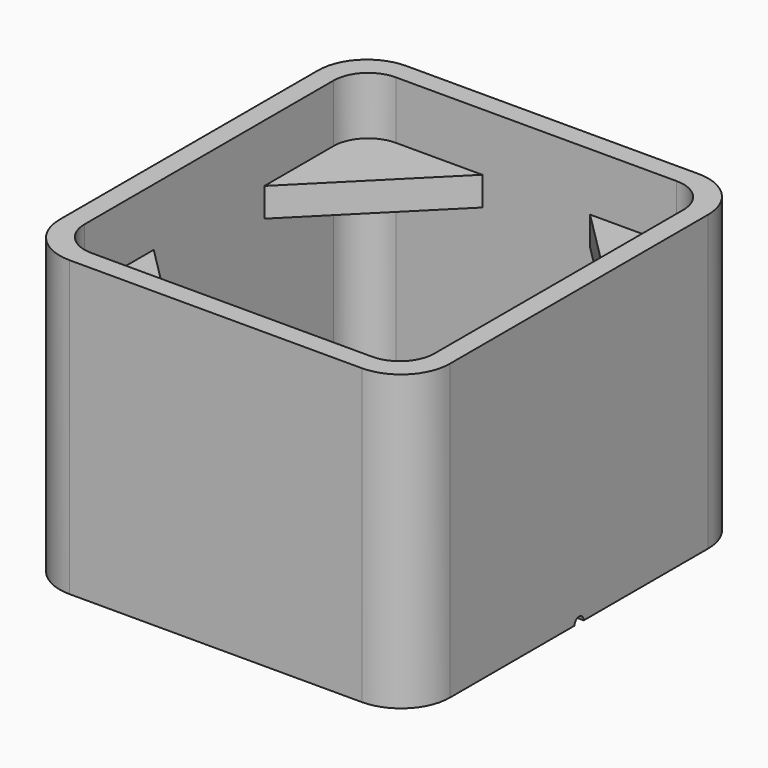
from build123d import *

# Parameters (mm, degrees)
F1_DEPTH = 3
F3_DEPTH = 38
F5_DEPTH = 5
F7_DEPTH = 10
F9_DEPTH = 67.701


# Not quite as in the source:
# - a feature names something its author has since deleted; it is built from what else it names


with BuildPart() as f1:
    # F0 (on Top) → F1 (new body)
    with BuildSketch(Plane.XY):
        with BuildLine():
            Line((-25.35, -36.5), (25.35, -36.5))
            ThreePointArc((25.35, -36.5), (31.3604076401, -34.0104076401), (33.85, -28))
            Line((33.85, -28), (33.85, 28))
            ThreePointArc((33.85, 28), (31.3604076401, 34.0104076401), (25.35, 36.5))
            Line((25.35, 36.5), (-25.35, 36.5))
            ThreePointArc((-25.35, 36.5), (-31.3604076401, 34.0104076401), (-33.85, 28))
            Line((-33.85, 28), (-33.85, -28))
            ThreePointArc((-33.85, -28), (-31.3604076401, -34.0104076401), (-25.35, -36.5))
        make_face()
    extrude(amount=F1_DEPTH)

    # F2 (on face) → F3 (join)
    with BuildSketch(Plane.XY.offset(3)):
        with BuildLine():
            ThreePointArc((-25.35, 36.5), (-31.3604076401, 34.0104076401), (-33.85, 28))
            Line((-33.85, 28), (-33.85, -28))
            ThreePointArc((-33.85, -28), (-31.3604076401, -34.0104076401), (-25.35, -36.5))
            Line((-25.35, -36.5), (25.35, -36.5))
            ThreePointArc((25.35, -36.5), (31.3604076401, -34.0104076401), (33.85, -28))
            Line((33.85, -28), (33.85, 28))
            ThreePointArc((33.85, 28), (31.3604076401, 34.0104076401), (25.35, 36.5))
            Line((25.35, 36.5), (-25.35, 36.5))
        make_face()
        with BuildLine():
            ThreePointArc((30.35, -27), (28.5926406871, -31.2426406871), (24.35, -33))
            Line((24.35, -33), (-24.35, -33))
            ThreePointArc((-24.35, -33), (-28.5926406871, -31.2426406871), (-30.35, -27))
            Line((-30.35, -27), (-30.35, 27))
            ThreePointArc((-30.35, 27), (-28.5926406871, 31.2426406871), (-24.35, 33))
            Line((-24.35, 33), (24.35, 33))
            ThreePointArc((24.35, 33), (28.5926406871, 31.2426406871), (30.35, 27))
            Line((30.35, 27), (30.35, -27))
        make_face(mode=Mode.SUBTRACT)
    extrude(amount=F3_DEPTH)

    # F4 (on face) → F5 (join)
    with BuildSketch(Plane.XY.offset(41)):
        with BuildLine():
            Line((25.35, 36.5), (-25.35, 36.5))
            ThreePointArc((-25.35, 36.5), (-31.3604076401, 34.0104076401), (-33.85, 28))
            Line((-33.85, 28), (-33.85, -28))
            ThreePointArc((-33.85, -28), (-31.3604076401, -34.0104076401), (-25.35, -36.5))
            Line((-25.35, -36.5), (25.35, -36.5))
            ThreePointArc((25.35, -36.5), (31.3604076401, -34.0104076401), (33.85, -28))
            Line((33.85, -28), (33.85, 28))
            ThreePointArc((33.85, 28), (31.3604076401, 34.0104076401), (25.35, 36.5))
        make_face()
        Polygon((24.35, 33), (30.35, 33), (30.35, 27), (30.35, 12), (30.35, -12), (30.35, -27), (30.35, -33), (24.35, -33), (9.35, -33), (-9.35, -33), (-24.35, -33), (-30.35, -33), (-30.35, -27), (-30.35, -12), (-30.35, 12), (-30.35, 27), (-30.35, 33), (-24.35, 33), (-9.35, 33), (9.35, 33), align=None, mode=Mode.SUBTRACT)
        with BuildLine():
            ThreePointArc((-30.35, 27), (-28.5926406871, 31.2426406871), (-24.35, 33))
            Line((-24.35, 33), (-30.35, 33))
            Line((-30.35, 33), (-30.35, 27))
        make_face()
        with BuildLine():
            Line((30.35, 27), (30.35, 33))
            Line((30.35, 33), (24.35, 33))
            ThreePointArc((24.35, 33), (28.5926406871, 31.2426406871), (30.35, 27))
        make_face()
        with BuildLine():
            Line((30.35, -33), (30.35, -27))
            ThreePointArc((30.35, -27), (28.5926406871, -31.2426406871), (24.35, -33))
            Line((24.35, -33), (30.35, -33))
        make_face()
        with BuildLine():
            ThreePointArc((-24.35, -33), (-28.5926406871, -31.2426406871), (-30.35, -27))
            Line((-30.35, -27), (-30.35, -33))
            Line((-30.35, -33), (-24.35, -33))
        make_face()
        with BuildLine():
            Line((30.35, -27), (30.35, -12))
            Line((30.35, -12), (9.35, -33))
            Line((9.35, -33), (24.35, -33))
            ThreePointArc((24.35, -33), (28.5926406871, -31.2426406871), (30.35, -27))
        make_face()
        with BuildLine():
            ThreePointArc((30.35, 27), (28.5926406871, 31.2426406871), (24.35, 33))
            Line((24.35, 33), (9.35, 33))
            Line((9.35, 33), (30.35, 12))
            Line((30.35, 12), (30.35, 27))
        make_face()
        with BuildLine():
            Line((-30.35, 12), (-9.35, 33))
            Line((-9.35, 33), (-24.35, 33))
            ThreePointArc((-24.35, 33), (-28.5926406871, 31.2426406871), (-30.35, 27))
            Line((-30.35, 27), (-30.35, 12))
        make_face()
        with BuildLine():
            Line((-9.35, -33), (-30.35, -12))
            Line((-30.35, -12), (-30.35, -27))
            ThreePointArc((-30.35, -27), (-28.5926406871, -31.2426406871), (-24.35, -33))
            Line((-24.35, -33), (-9.35, -33))
        make_face()
    extrude(amount=-F5_DEPTH)

    # F6 (on face) → F7 (join)
    with BuildSketch(Plane.XY.offset(41)):
        with BuildLine():
            Line((25.35, 36.5), (-25.35, 36.5))
            ThreePointArc((-25.35, 36.5), (-31.3604076401, 34.0104076401), (-33.85, 28))
            Line((-33.85, 28), (-33.85, -28))
            ThreePointArc((-33.85, -28), (-31.3604076401, -34.0104076401), (-25.35, -36.5))
            Line((-25.35, -36.5), (25.35, -36.5))
            ThreePointArc((25.35, -36.5), (31.3604076401, -34.0104076401), (33.85, -28))
            Line((33.85, -28), (33.85, 28))
            ThreePointArc((33.85, 28), (31.3604076401, 34.0104076401), (25.35, 36.5))
        make_face()
        with BuildLine():
            Line((9.35, 33), (24.35, 33))
            ThreePointArc((24.35, 33), (28.5926406871, 31.2426406871), (30.35, 27))
            Line((30.35, 27), (30.35, 12))
            Line((30.35, 12), (30.35, -12))
            Line((30.35, -12), (30.35, -27))
            ThreePointArc((30.35, -27), (28.5926406871, -31.2426406871), (24.35, -33))
            Line((24.35, -33), (9.35, -33))
            Line((9.35, -33), (-9.35, -33))
            Line((-9.35, -33), (-24.35, -33))
            ThreePointArc((-24.35, -33), (-28.5926406871, -31.2426406871), (-30.35, -27))
            Line((-30.35, -27), (-30.35, -12))
            Line((-30.35, -12), (-30.35, 12))
            Line((-30.35, 12), (-30.35, 27))
            ThreePointArc((-30.35, 27), (-28.5926406871, 31.2426406871), (-24.35, 33))
            Line((-24.35, 33), (-9.35, 33))
            Line((-9.35, 33), (9.35, 33))
        make_face(mode=Mode.SUBTRACT)
    extrude(amount=F7_DEPTH)

    # F8 (on face) → F9 (cut, through all)
    with BuildSketch(Plane.YZ.offset(33.85)):
        with BuildLine():
            Line((-1, 0), (1, 0))
            ThreePointArc((1, 0), (0, 1), (-1, 0))
        make_face()
    extrude(amount=-F9_DEPTH, mode=Mode.SUBTRACT)


solid = f1.part
